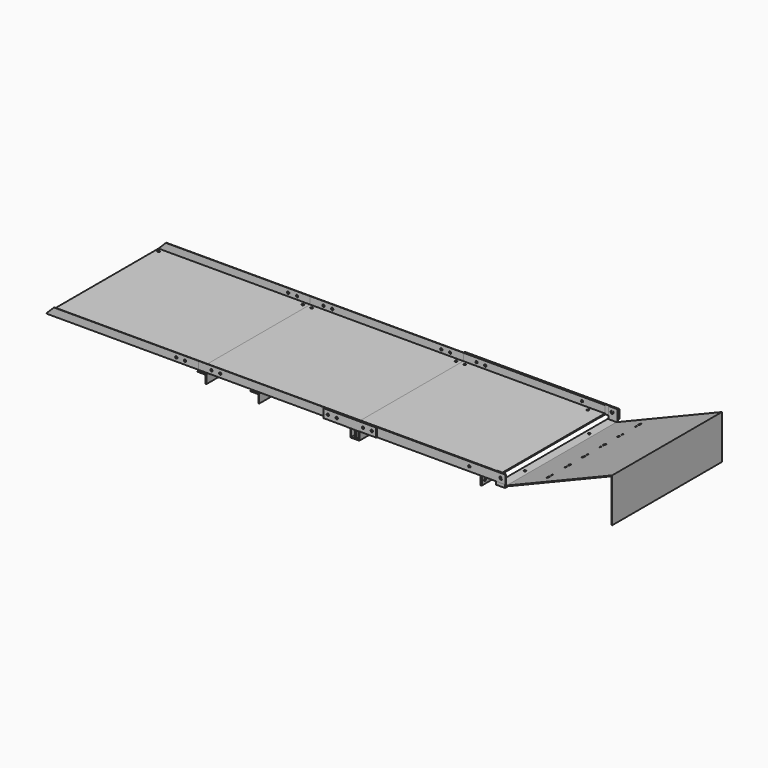
from build123d import *

# Parameters (mm, degrees)
F1_DEPTH       = 780
F3_DEPTH       = 50
F4_R           = 8.5
F5_DEPTH       = 802.001
F6_W           = 880
F6_H           = 50
F7_DEPTH       = 4
F8_W           = 805
F8_H           = 4
F9_DEPTH       = 46
F10_W          = 880
F10_H          = 50
F11_DEPTH      = 4
F12_W          = 805
F12_H          = 4
F13_DEPTH      = 46
F14_W          = 50
F14_H          = 870
F15_DEPTH      = 4
F16_W          = 4
F16_H          = 870
F17_DEPTH      = 46
F18_W          = 4
F18_H          = 870
F19_DEPTH      = 44
F20_W          = 4
F20_H          = 870
F21_DEPTH      = 46
F22_R          = 8.5
F23_DEPTH      = 870.001
F25_R          = 8.5
F26_DEPTH      = 64.001
F27_R          = 8.5
F27_R_2        = 5.75
F28_DEPTH      = 262.7725410792
F29_R          = 6
F30_DEPTH      = 254.001
F31_R          = 6.5
F32_DEPTH      = 38.001
F33_W          = 50
F33_H          = 50
F33_W_2        = 42
F33_H_2        = 42
F34_DEPTH      = 810
F36_W          = 300
F36_H          = 50
F36_R          = 6.5
F36_W_2        = 150
F37_DEPTH      = 5
F38_R          = 6.5
F39_DEPTH      = 870.001
F40_R          = 6.5
F41_DEPTH      = 815.001
F42_R          = 6.5
F43_DEPTH      = 25
F44_R          = 6.5
F45_DEPTH      = 350.001
F50_R          = 6.5
F51_DEPTH      = 25
F54_DEPTH      = 350.001
F57_DEPTH      = 50.001
F52_R          = 6.5
F58_DEPTH      = 25
F59_R          = 6.5
F60_DEPTH      = 25
F61_R          = 6.5
F62_DEPTH      = 25
F63_R          = 6.5
F64_DEPTH      = 25
F65_R          = 6.5
F66_DEPTH      = 25
F67_R          = 6.5
F68_DEPTH      = 25
F69_W          = 805
F69_H          = 753.5
F69_R          = 6.5
F69_H_2        = 44.5
F70_DEPTH      = 2.5
F71_W          = 805
F71_H          = 2.5
F72_DEPTH      = 42
F73_R          = 6.5
F74_DEPTH      = 64.001
F74_DEPTH_BACK = 811.001
F75_DEPTH      = 870
F76_R          = 3.181790525
F76_R_2        = 6.5
F77_DEPTH      = 864.501
F78_R          = 4.6535428545
F78_R_2        = 6.5
F78_R_3        = 3.6492006741
F79_DEPTH      = 25
F82_DEPTH      = 864.501
F81_R          = 6.5
F83_DEPTH      = 2.5
F84_R          = 6.5
F85_DEPTH      = 2.5


with BuildPart() as f1:
    # F0 (on Front) → F1 (new body)
    with BuildSketch(Plane.XZ):
        Polygon((0, 4), (0, 0), (50.7881634193, 0), (646, 244.0368529981), (646, 0), (650, 0), (650, 250), (50, 4), align=None)
    extrude(amount=-F1_DEPTH)

    # F25 (on face) → F26 (cut, through all)
    with BuildSketch(Plane.XZ.offset(-791)):
        with Locations((30, 41)):
            Circle(F25_R)
    extrude(amount=-F26_DEPTH, mode=Mode.SUBTRACT)

    # F27 (on face) → F28 (cut, through all)
    with BuildSketch(Plane(origin=(5.7914562109, 0, -14.1255029535), x_dir=(0.9252519052, 0, 0.3793532811), z_dir=(-0.3793532811, 0, 0.9252519052))):
        with Locations((247.780008385, 715)):
            Circle(F27_R)
        with Locations((247.780008385, 565)):
            Circle(F27_R)
        with Locations((247.780008385, 465)):
            Circle(F27_R)
        with Locations((247.780008385, 315)):
            Circle(F27_R)
        with Locations((247.780008385, 215)):
            Circle(F27_R)
        with Locations((247.780008385, 65)):
            Circle(F27_R)
        with Locations((247.780008385, 688)):
            Circle(F27_R_2)
        with Locations((247.780008385, 592)):
            Circle(F27_R_2)
        with Locations((247.780008385, 438)):
            Circle(F27_R_2)
        with Locations((247.780008385, 342)):
            Circle(F27_R_2)
        with Locations((247.780008385, 188)):
            Circle(F27_R_2)
        with Locations((247.780008385, 92)):
            Circle(F27_R_2)
    extrude(amount=-F28_DEPTH, mode=Mode.SUBTRACT)


with BuildPart() as f3:
    # F2 (on Right) → F3 (new body)
    with BuildSketch(Plane.YZ):
        Polygon((787, 0), (0, 0), (-7, 0), (-7, 66), (-11, 66), (-11, -4), (791, -4), (791, 66), (787, 66), align=None)
    extrude(amount=F3_DEPTH)

    # F4 (on face) → F5 (cut, through all)
    with BuildSketch(Plane.XZ.offset(11)):
        with Locations((20, 41)):
            Circle(F4_R)
    extrude(amount=-F5_DEPTH, mode=Mode.SUBTRACT)


with BuildPart() as f7:
    # F6 (on face) → F7 (new body)
    with BuildSketch(Plane.XZ.offset(11)):
        with Locations((-385, 41)):
            Rectangle(F6_W, F6_H)
    extrude(amount=F7_DEPTH)

    # F8 (on face) → F9 (join)
    with BuildSketch(Plane(origin=(0, -11, 0), x_dir=(-1, 0, 0), z_dir=(0, 1, 0))):
        with Locations((422.5, 18)):
            Rectangle(F8_W, F8_H)
    extrude(amount=F9_DEPTH)


with BuildPart() as f11:
    # F10 (on face) → F11 (new body)
    with BuildSketch(Plane(origin=(0, 791, 0), x_dir=(-1, 0, 0), z_dir=(0, 1, 0))):
        with Locations((385, 41)):
            Rectangle(F10_W, F10_H)
    extrude(amount=F11_DEPTH)

    # F12 (on face) → F13 (join)
    with BuildSketch(Plane.XZ.offset(-791)):
        with Locations((-422.5, 18)):
            Rectangle(F12_W, F12_H)
    extrude(amount=F13_DEPTH)


with BuildPart() as f15:
    # F14 (on face) → F15 (new body)
    with BuildSketch(Plane(origin=(0, 0, 16), x_dir=(1, 0, 0), z_dir=(0, 0, -1))):
        with Locations((-820, -420)):
            Rectangle(F14_W, F14_H)
    extrude(amount=F15_DEPTH)

    # F18 (on face) → F19 (join)
    with BuildSketch(Plane(origin=(0, 0, 12), x_dir=(1, 0, 0), z_dir=(0, 0, -1))):
        with Locations((-797, -420)):
            Rectangle(F18_W, F18_H)
    extrude(amount=F19_DEPTH)


with BuildPart() as f15b:
    # F14 (on face) → F15, piece 2 (new body)
    with BuildSketch(Plane(origin=(0, 0, 16), x_dir=(1, 0, 0), z_dir=(0, 0, -1))):
        with Locations((-1670, -420)):
            Rectangle(F14_W, F14_H)
    extrude(amount=F15_DEPTH)

    # F16 (on face) → F17 (join)
    with BuildSketch(Plane(origin=(0, 0, 12), x_dir=(1, 0, 0), z_dir=(0, 0, -1))):
        with Locations((-1647, -420)):
            Rectangle(F16_W, F16_H)
    extrude(amount=F17_DEPTH)


with BuildPart() as f15c:
    # F14 (on face) → F15, piece 3 (new body)
    with BuildSketch(Plane(origin=(0, 0, 16), x_dir=(1, 0, 0), z_dir=(0, 0, -1))):
        with Locations((-60.1201042533, -420)):
            Rectangle(F14_W, F14_H)
    extrude(amount=F15_DEPTH)

    # F20 (on face) → F21 (join)
    with BuildSketch(Plane(origin=(0, 0, 12), x_dir=(1, 0, 0), z_dir=(0, 0, -1))):
        with Locations((-83.1201042533, -420)):
            Rectangle(F20_W, F20_H)
    extrude(amount=F21_DEPTH)

    # F50 (on face) → F51 (cut)
    with BuildSketch(Plane.XY.offset(16)):
        with Locations((-60.1201042533, 780)):
            Circle(F50_R)
        with Locations((-60.1201042533, 730)):
            Circle(F50_R)
    extrude(amount=-F51_DEPTH, mode=Mode.SUBTRACT)

    # F56 (on face) → F57 (cut, through all)
    with BuildSketch(Plane.XY.offset(16)):
        Polygon((-35.1201042533, -15), (-35.1201042533, 35), (-85.1201042533, -15), align=None)
    extrude(amount=-F57_DEPTH, mode=Mode.SUBTRACT)

    # F67 (on face) → F68 (cut)
    with BuildSketch(Plane.YZ.offset(-81.1201042533)):
        with Locations((830, -14)):
            Circle(F67_R)
        with Locations((10, -14)):
            Circle(F67_R)
    extrude(amount=-F68_DEPTH, mode=Mode.SUBTRACT)


with BuildPart() as f23_tool:
    # F22 (on face) → F23 (new body, through all)
    with BuildSketch(Plane.XZ.offset(15)):
        with Locations((30, 41)):
            Circle(F22_R)
    extrude(amount=-F23_DEPTH)


with BuildPart() as f7_1:
    add(f7.part)

    # F23: cut by f23_tool
    add(f23_tool.part, mode=Mode.SUBTRACT)


with BuildPart() as f11_1:
    add(f11.part)

    # F23: cut by f23_tool
    add(f23_tool.part, mode=Mode.SUBTRACT)


with BuildPart() as f30_tool:
    # F29 (on face) → F30 (new body, through all)
    with BuildSketch(Plane(origin=(0, 0, -4), x_dir=(1, 0, 0), z_dir=(0, 0, -1))):
        with Locations((25, -619)):
            Circle(F29_R)
        with Locations((25, -161)):
            Circle(F29_R)
    extrude(amount=-F30_DEPTH)


with BuildPart() as f1_1:
    add(f1.part)

    # F30: cut by f30_tool
    add(f30_tool.part, mode=Mode.SUBTRACT)

    # F31 (on face) → F32 (cut, through all)
    with BuildSketch(Plane.XY.offset(4)):
        with Locations((25, 619)):
            Circle(F31_R)
        with Locations((25, 161)):
            Circle(F31_R)
    extrude(amount=-F32_DEPTH, mode=Mode.SUBTRACT)

    # F40 (on face) → F41 (cut, through all)
    with BuildSketch(Plane(origin=(0, 795, 0), x_dir=(-1, 0, 0), z_dir=(0, 1, 0))):
        with Locations((700, 41)):
            Circle(F40_R)
        with Locations((750, 41)):
            Circle(F40_R)
    extrude(amount=-F41_DEPTH, mode=Mode.SUBTRACT)


with BuildPart() as f3_1:
    add(f3.part)

    # F30: cut by f30_tool
    add(f30_tool.part, mode=Mode.SUBTRACT)


with BuildPart() as f34:
    # F33 (on face) → F34 (new body)
    with BuildSketch(Plane.XZ.offset(15)):
        with Locations((-800, -9)):
            Rectangle(F33_W, F33_H)
        with Locations((-800, -9)):
            Rectangle(F33_W_2, F33_H_2, mode=Mode.SUBTRACT)
    extrude(amount=-F34_DEPTH)

    # F52 (on face) → F58 (cut)
    with BuildSketch(Plane.XY.offset(16)):
        with Locations((-800, 765)):
            Circle(F52_R)
        with Locations((-800, 15)):
            Circle(F52_R)
    extrude(amount=-F58_DEPTH, mode=Mode.SUBTRACT)


with BuildPart() as f35_1:
    # F35: copy of F15b
    add(f15b.part.moved(Location((300, 0, 0))))

    # F44 (on face) → F45 (cut, through all)
    with BuildSketch(Plane.YZ.offset(-1345)):
        with Locations((60, -9)):
            Circle(F44_R)
        with Locations((110, -9)):
            Circle(F44_R)
    extrude(amount=-F45_DEPTH, mode=Mode.SUBTRACT)


with BuildPart() as f37:
    # F36 (on face) → F37 (new body)
    with BuildSketch(Plane.XZ.offset(15)):
        with Locations((-825, 41)):
            Rectangle(F36_W, F36_H)
        with Locations((-950, 41)):
            Circle(F36_R, mode=Mode.SUBTRACT)
        with Locations((-900, 41)):
            Circle(F36_R, mode=Mode.SUBTRACT)
        with Locations((-750, 41)):
            Circle(F36_R, mode=Mode.SUBTRACT)
        with Locations((-700, 41)):
            Circle(F36_R, mode=Mode.SUBTRACT)
        with Locations((-900, 41)):
            Rectangle(F36_W_2, F36_H)
        with Locations((-950, 41)):
            Circle(F36_R, mode=Mode.SUBTRACT)
        with Locations((-900, 41)):
            Circle(F36_R, mode=Mode.SUBTRACT)
    extrude(amount=F37_DEPTH)


with BuildPart() as f39_tool:
    # F38 (on face) → F39 (new body, through all)
    with BuildSketch(Plane.XZ.offset(15)):
        with Locations((-750, 41)):
            Circle(F38_R)
        with Locations((-700, 41)):
            Circle(F38_R)
    extrude(amount=-F39_DEPTH)


with BuildPart() as f7_2:
    add(f7_1.part)

    # F39: cut by f39_tool
    add(f39_tool.part, mode=Mode.SUBTRACT)

    # F59 (on face) → F60 (cut)
    with BuildSketch(Plane.XY.offset(20)):
        with Locations((-100, 15)):
            Circle(F59_R)
        with Locations((-800, 15)):
            Circle(F59_R)
    extrude(amount=-F60_DEPTH, mode=Mode.SUBTRACT)


with BuildPart() as f11_2:
    add(f11_1.part)

    # F39: cut by f39_tool
    add(f39_tool.part, mode=Mode.SUBTRACT)

    # F61 (on face) → F62 (cut)
    with BuildSketch(Plane.XY.offset(20)):
        with Locations((-100, 765)):
            Circle(F61_R)
        with Locations((-800, 765)):
            Circle(F61_R)
    extrude(amount=-F62_DEPTH, mode=Mode.SUBTRACT)


with BuildPart() as f15b_1:
    add(f15b.part)

    # F42 (on face) → F43 (cut)
    with BuildSketch(Plane.YZ.offset(-1645)):
        with Locations((60, -9)):
            Circle(F42_R)
        with Locations((110, -9)):
            Circle(F42_R)
        with Locations((780, -9)):
            Circle(F42_R)
        with Locations((730, -9)):
            Circle(F42_R)
    extrude(amount=-F43_DEPTH, mode=Mode.SUBTRACT)

    # F63 (on face) → F64 (cut)
    with BuildSketch(Plane(origin=(0, 0, 12), x_dir=(1, 0, 0), z_dir=(0, 0, -1))):
        with Locations((-1675, -830)):
            Circle(F63_R)
        with Locations((-1675, -10)):
            Circle(F63_R)
    extrude(amount=-F64_DEPTH, mode=Mode.SUBTRACT)


with BuildPart() as f46_1:
    # F46: copy of F35_1
    add(f35_1.part.moved(Location((150, 0, 0))))


with BuildPart() as f47_1:
    # F47: copy of F35_1
    add(f35_1.part.moved(Location((250, 0, 0))))


with BuildPart() as f35_1_1:
    add(f35_1.part)

    # F53 (on face) → F54 (cut, through all)
    with BuildSketch(Plane.YZ.offset(-1345)):
        Polygon((855, -34), (855, 16), (805, -34), align=None)
    extrude(amount=-F54_DEPTH, mode=Mode.SUBTRACT)

    # F65 (on face) → F66 (cut)
    with BuildSketch(Plane(origin=(0, 0, 12), x_dir=(1, 0, 0), z_dir=(0, 0, -1))):
        with Locations((-1375, -830)):
            Circle(F65_R)
        with Locations((-1375, -10)):
            Circle(F65_R)
    extrude(amount=-F66_DEPTH, mode=Mode.SUBTRACT)


with BuildPart() as f70:
    # F69 (on face) → F70 (new body)
    with BuildSketch(Plane.XY.offset(20)):
        with Locations((-422.5, 411.75)):
            Rectangle(F69_W, F69_H)
        with Locations((-800, 765)):
            Circle(F69_R, mode=Mode.SUBTRACT)
        with Locations((-100, 765)):
            Circle(F69_R, mode=Mode.SUBTRACT)
        with Locations((-422.5, 12.75)):
            Rectangle(F69_W, F69_H_2)
        with Locations((-800, 15)):
            Circle(F69_R, mode=Mode.SUBTRACT)
        with Locations((-100, 15)):
            Circle(F69_R, mode=Mode.SUBTRACT)
    extrude(amount=F70_DEPTH)

    # F71 (on face) → F72 (join)
    with BuildSketch(Plane.XY.offset(22.5)):
        with Locations((-422.5, -8.25)):
            Rectangle(F71_W, F71_H)
        with Locations((-422.5, 787.25)):
            Rectangle(F71_W, F71_H)
    extrude(amount=F72_DEPTH)


with BuildPart() as f74_tool:
    # F73 (on face) → F74 (new body, two sides)
    with BuildSketch(Plane.XZ.offset(-791)) as f74_sk:
        with Locations((-750, 41)):
            Circle(F73_R)
        with Locations((-700, 41)):
            Circle(F73_R)
        with Locations((-150, 41)):
            Circle(F73_R)
    extrude(amount=-F74_DEPTH)
    extrude(f74_sk.sketch, amount=F74_DEPTH_BACK)


with BuildPart() as f7_3:
    add(f7_2.part)

    # F74: cut by f74_tool
    add(f74_tool.part, mode=Mode.SUBTRACT)


with BuildPart() as f11_3:
    add(f11_2.part)

    # F74: cut by f74_tool
    add(f74_tool.part, mode=Mode.SUBTRACT)


with BuildPart() as f70_1:
    add(f70.part)

    # F74: cut by f74_tool
    add(f74_tool.part, mode=Mode.SUBTRACT)


with BuildPart() as f75:
    # F75 (new): a face of the model
    f75_faces = [f70_1.part.faces().sort_by_distance(p)[0] for p in [
        (-825, 787.7007602049, 42.25),
    ]]
    extrude(f75_faces, amount=F75_DEPTH)

    # F76 (on face) → F77 (cut, through all)
    with BuildSketch(Plane.XZ.offset(9.5)):
        with Locations((-750, 41)):
            Circle(F76_R)
        with Locations((-950, 41)):
            Circle(F76_R_2)
        with Locations((-900, 41)):
            Circle(F76_R_2)
        with Locations((-1570, 41)):
            Circle(F76_R_2)
        with Locations((-1620, 41)):
            Circle(F76_R_2)
    extrude(amount=-F77_DEPTH, mode=Mode.SUBTRACT)

    # F78 (on face) → F79 (cut)
    with BuildSketch(Plane.XY.offset(22.5)):
        with Locations((-800, 765)):
            Circle(F78_R)
        with Locations((-850, 765)):
            Circle(F78_R_2)
        with Locations((-1670, 765)):
            Circle(F78_R_2)
        with Locations((-800, 15)):
            Circle(F78_R_3)
        with Locations((-850, 15)):
            Circle(F78_R_2)
        with Locations((-1670, 15)):
            Circle(F78_R_2)
    extrude(amount=-F79_DEPTH, mode=Mode.SUBTRACT)


with BuildPart() as f80_1:
    # F80: copy of F75
    add(f75.part.moved(Location((-870, 0, 0))))

    # F81 (on face) → F82 (cut, through all)
    with BuildSketch(Plane.XZ.offset(9.5)):
        Polygon((-2560, 20), (-2515.5, 64.5), (-2565, 64.5), (-2565, 20), align=None)
    extrude(amount=-F82_DEPTH, mode=Mode.SUBTRACT)

    # F81 (on face) → F83 (join)
    with BuildSketch(Plane.XZ.offset(9.5)):
        with Locations((-2490, 41)):
            Circle(F81_R)
        with Locations((-2440, 41)):
            Circle(F81_R)
    extrude(amount=-F83_DEPTH)

    # F84 (on face) → F85 (join)
    with BuildSketch(Plane.XZ.offset(-786)):
        with Locations((-2490, 41)):
            Circle(F84_R)
        with Locations((-2440, 41)):
            Circle(F84_R)
    extrude(amount=-F85_DEPTH)


solid = Compound([f15.part, f15c.part, f1_1.part, f3_1.part, f34.part, f37.part, f15b_1.part, f35_1_1.part, f7_3.part, f11_3.part, f70_1.part, f75.part, f80_1.part])
